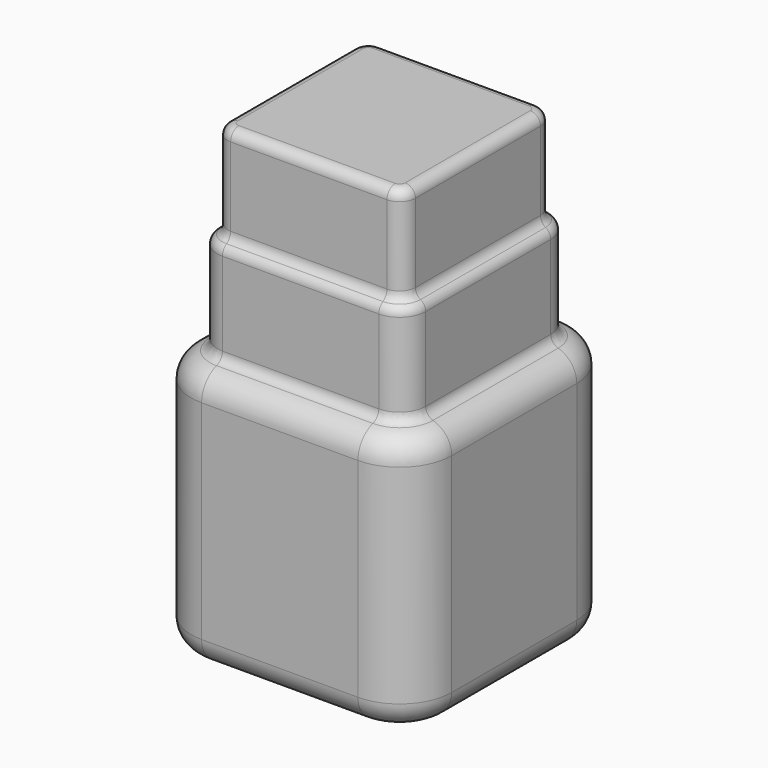
from build123d import *

# Parameters (mm, degrees)
F0_W     = 127
F0_H     = 127
F1_DEPTH = 127
F2_R     = 25.4
F3_R     = 12.7
F4_DEPTH = 50
F5_R     = 5
F6_DEPTH = 47
F7_R     = 5


# Not quite as in the source:
# - two fillets or chamfers of one size are made in one step


with BuildPart() as f1:
    # F0 (on Front) → F1 (new body)
    with BuildSketch(Plane.XZ):
        Rectangle(F0_W, F0_H)
    extrude(amount=F1_DEPTH)

    # F2
    f2_edges = [f1.edges().sort_by_distance(p)[0] for p in [
        (-63.5, -127, 0),
        (63.5, -127, 0),
        (-63.5, 0, 0),
        (63.5, 0, 0),
    ]]
    fillet(f2_edges, radius=F2_R)

    # F3
    f3_edges = [f1.edges().sort_by_distance(p)[0] for p in [
        (-63.5, -63.5, 63.5),
        (0, -127, -63.5),
        (63.5, -63.5, -63.5),
        (56.060512, -7.439488, -63.5),
        (56.060512, -119.560512, -63.5),
        (0, 0, -63.5),
        (-56.060512, -7.439488, -63.5),
        (-56.060512, -119.560512, -63.5),
        (-63.5, -63.5, -63.5),
    ]]
    fillet(f3_edges, radius=F3_R)

    # F4 (add): a face of the model
    f4_faces = [f1.faces().sort_by_distance(p)[0] for p in [
        (0, -63.5, 63.5),
    ]]
    extrude(f4_faces, amount=F4_DEPTH)

    # F5
    f5_edges = [f1.edges().sort_by_distance(p)[0] for p in [
        (-50.8, -63.5, 63.5),
        (-47.080256, -16.419744, 63.5),
        (-50.8, -63.5, 113.5),
        (-47.080256, -110.580256, 63.5),
        (0, -12.7, 63.5),
        (-47.080256, -16.419744, 113.5),
        (-47.080256, -110.580256, 113.5),
        (0, -12.7, 113.5),
        (0, -114.3, 113.5),
        (47.080256, -16.419744, 113.5),
        (47.080256, -110.580256, 113.5),
        (50.8, -63.5, 113.5),
        (0, -114.3, 63.5),
        (47.080256, -16.419744, 63.5),
        (47.080256, -110.580256, 63.5),
        (50.8, -63.5, 63.5),
    ]]
    fillet(f5_edges, radius=F5_R)

    # F6 (add): a face of the model
    f6_faces = [f1.faces().sort_by_distance(p)[0] for p in [
        (0, -63.5, 113.5),
    ]]
    extrude(f6_faces, amount=F6_DEPTH)

    # F7
    f7_edges = [f1.edges().sort_by_distance(p)[0] for p in [
        (-45.8, -63.5, 113.5),
        (-43.544722, -19.955278, 113.5),
        (-45.8, -63.5, 160.5),
        (-43.544722, -107.044722, 113.5),
        (0, -17.7, 113.5),
        (-43.544722, -19.955278, 160.5),
        (-43.544722, -107.044722, 160.5),
        (0, -17.7, 160.5),
        (0, -109.3, 160.5),
        (43.544722, -19.955278, 160.5),
        (43.544722, -107.044722, 160.5),
        (45.8, -63.5, 160.5),
        (0, -109.3, 113.5),
        (43.544722, -19.955278, 113.5),
        (43.544722, -107.044722, 113.5),
        (45.8, -63.5, 113.5),
    ]]
    fillet(f7_edges, radius=F7_R)


solid = f1.part
